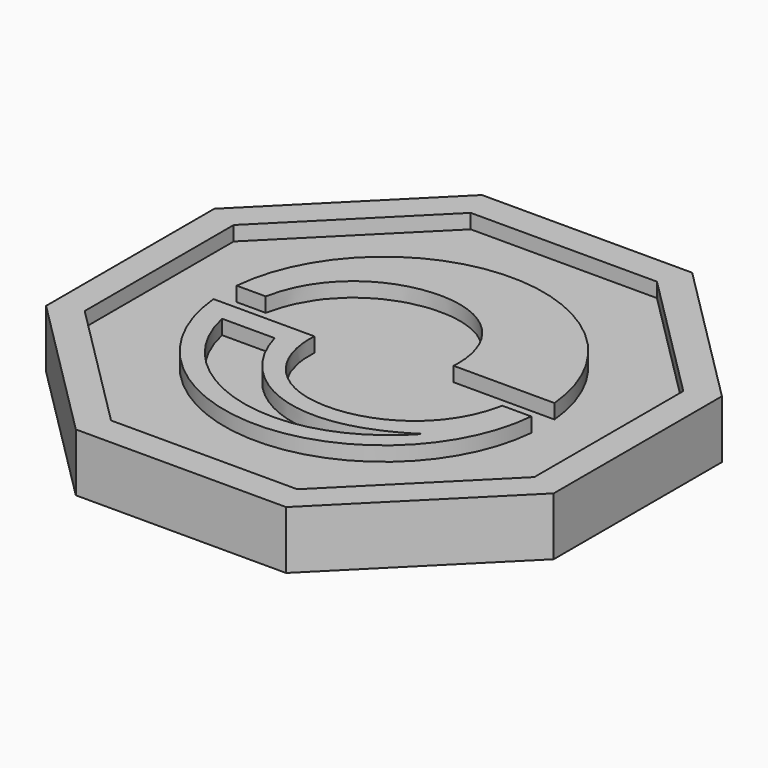
from build123d import *

# Parameters (mm, degrees)
F1_DEPTH = 2
F2_DEPTH = 1.5


# Not quite as in the source:
# - a feature names something its author has since deleted; it is built from what else it names


with BuildPart() as f1:
    # F0 (on Top) → F1 (new body)
    with BuildSketch(Plane.XY):
        with BuildLine():
            ThreePointArc((5.4772255751, 0.5), (0, 5.5), (-5.4772255751, 0.5))
            Line((-5.4772255751, 0.5), (-4.4772255751, 0.5))
            add(Edge.make_bspline(
                [(-4.4772255751, 0.5), (-3.9824196137, 2.9745399952), (0.3355675447, 4.4637305093), (2.0776381716, 1.8807736924), (2, 0.5)],
                knots=[0, 0, 0, 0, 0.5520438293, 1, 1, 1, 1], degree=3))
            Line((2, 0.5), (5.4772255751, 0.5))
        make_face()
    extrude(amount=F1_DEPTH)


with BuildPart() as f1b:
    # F0 (on Top) → F1, piece 2 (new body)
    with BuildSketch(Plane.XY):
        with BuildLine():
            Line((-2, -0.5), (-5.4772255751, -0.5))
            ThreePointArc((-5.4772255751, -0.5), (0, -5.5), (5.4772255751, -0.5))
            Line((5.4772255751, -0.5), (4.4772255751, -0.5))
            add(Edge.make_bspline(
                [(4.4772255751, -0.5), (3.9824196137, -2.9745399952), (-0.3355675447, -4.4637305093), (-2.0776381716, -1.8807736924), (-2, -0.5)],
                knots=[0, 0, 0, 0, 0.5520438293, 1, 1, 1, 1], degree=3))
        make_face()
        with BuildLine():
            add(Edge.make_bspline(
                [(-4.582575695, -1.25), (-3.830221016, -4.746818915), (0.8803614764, -6.3501568511), (3.8508872967, -3.1061938498)],
                knots=[0, 0, 0, 0, 8.6353201238, 8.6353201238, 8.6353201238, 8.6353201238], degree=3))
            Line((-4.582575695, -1.25), (-2.770407591, -1.25))
            add(Edge.make_bspline(
                [(-2.770407591, -1.25), (-2.077735262, -3.7525005173), (0.7187846932, -5.1818331704), (3.8508872967, -3.1061938498)],
                knots=[0, 0, 0, 0, 6.876554486, 6.876554486, 6.876554486, 6.876554486], degree=3))
        make_face(mode=Mode.SUBTRACT)
    extrude(amount=F1_DEPTH)


with BuildPart() as f1c:
    # F0 (on Top) → F1, piece 3 (new body)
    with BuildSketch(Plane.XY):
        Polygon((3.6243686708, -8.75), (8.75, -3.6243686708), (8.75, 3.6243686708), (3.6243686708, 8.75), (-3.6243686708, 8.75), (-8.75, 3.6243686708), (-8.75, -3.6243686708), (-3.6243686708, -8.75), align=None)
        Polygon((7.75, 3.2101551084), (7.75, -3.2101551084), (3.2101551084, -7.75), (-3.2101551084, -7.75), (-7.75, -3.2101551084), (-7.75, 3.2101551084), (-3.2101551084, 7.75), (3.2101551084, 7.75), align=None, mode=Mode.SUBTRACT)
    extrude(amount=F1_DEPTH)


with BuildPart() as f2:
    # F0 (on Top) → F2 (new body)
    with BuildSketch(Plane.XY):
        with BuildLine():
            Line((-2.770407591, -1.25), (-4.582575695, -1.25))
            add(Edge.make_bspline(
                [(-4.582575695, -1.25), (-3.830221016, -4.746818915), (0.8803614764, -6.3501568511), (3.8508872967, -3.1061938498)],
                knots=[0, 0, 0, 0, 8.6353201238, 8.6353201238, 8.6353201238, 8.6353201238], degree=3))
            add(Edge.make_bspline(
                [(-2.770407591, -1.25), (-2.077735262, -3.7525005173), (0.7187846932, -5.1818331704), (3.8508872967, -3.1061938498)],
                knots=[0, 0, 0, 0, 6.876554486, 6.876554486, 6.876554486, 6.876554486], degree=3))
        make_face()
    extrude(amount=F2_DEPTH)


with BuildPart() as f2b:
    # F0 (on Top) → F2, piece 2 (new body)
    with BuildSketch(Plane.XY):
        Polygon((3.2101551084, -7.75), (7.75, -3.2101551084), (7.75, 3.2101551084), (3.2101551084, 7.75), (-3.2101551084, 7.75), (-7.75, 3.2101551084), (-7.75, -3.2101551084), (-3.2101551084, -7.75), align=None)
        with BuildLine():
            ThreePointArc((5.4772255751, -0.5), (0, -5.5), (-5.4772255751, -0.5))
            Line((-5.4772255751, -0.5), (-2, -0.5))
            add(Edge.make_bspline(
                [(4.4772255751, -0.5), (3.9824196137, -2.9745399952), (-0.3355675447, -4.4637305093), (-2.0776381716, -1.8807736924), (-2, -0.5)],
                knots=[0, 0, 0, 0, 0.5520438293, 1, 1, 1, 1], degree=3))
            Line((4.4772255751, -0.5), (5.4772255751, -0.5))
        make_face(mode=Mode.SUBTRACT)
        with BuildLine():
            Line((-4.4772255751, 0.5), (-5.4772255751, 0.5))
            ThreePointArc((-5.4772255751, 0.5), (0, 5.5), (5.4772255751, 0.5))
            Line((5.4772255751, 0.5), (2, 0.5))
            add(Edge.make_bspline(
                [(-4.4772255751, 0.5), (-3.9824196137, 2.9745399952), (0.3355675447, 4.4637305093), (2.0776381716, 1.8807736924), (2, 0.5)],
                knots=[0, 0, 0, 0, 0.5520438293, 1, 1, 1, 1], degree=3))
        make_face(mode=Mode.SUBTRACT)
    extrude(amount=F2_DEPTH)


solid = Compound([f1.part, f1b.part, f1c.part, f2.part, f2b.part])
